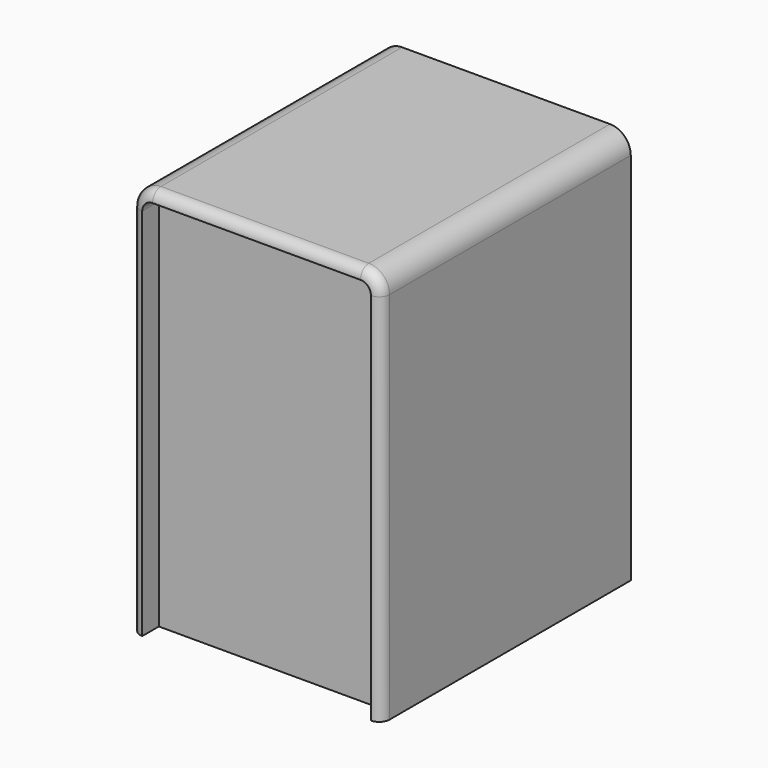
from build123d import *

# Parameters (mm, degrees)
F0_W     = 304.8
F0_H     = 381
F1_DEPTH = 482.6
F2_R     = 25.4
F3_R     = 12.7
F4_DEPTH = 25.4


# Not quite as in the source:
# - the program builds the solid bodies; features that only make, move or delete a surface that nothing else refers to are left out


with BuildPart() as f1:
    # F0 (on Top) → F1 (new body)
    with BuildSketch(Plane.XY):
        Rectangle(F0_W, F0_H)
    extrude(amount=F1_DEPTH)

    # F2
    f2_edges = [f1.edges().sort_by_distance(p)[0] for p in [
        (-152.4, 0, 482.6),
        (152.4, 0, 482.6),
    ]]
    fillet(f2_edges, radius=F2_R)

    # F3
    f3_edges = [f1.edges().sort_by_distance(p)[0] for p in [
        (-152.4, -190.5, 228.6),
        (-144.960512, -190.5, 475.160512),
        (0, -190.5, 482.6),
        (144.960512, -190.5, 475.160512),
        (152.4, -190.5, 228.6),
    ]]
    fillet(f3_edges, radius=F3_R)

    # F4 (cut): a face of the model
    f4_faces = [f1.faces().sort_by_distance(p)[0] for p in [
        (0, -190.5, 234.8275474118),
    ]]
    extrude(f4_faces, amount=-F4_DEPTH, mode=Mode.SUBTRACT)


solid = f1.part
